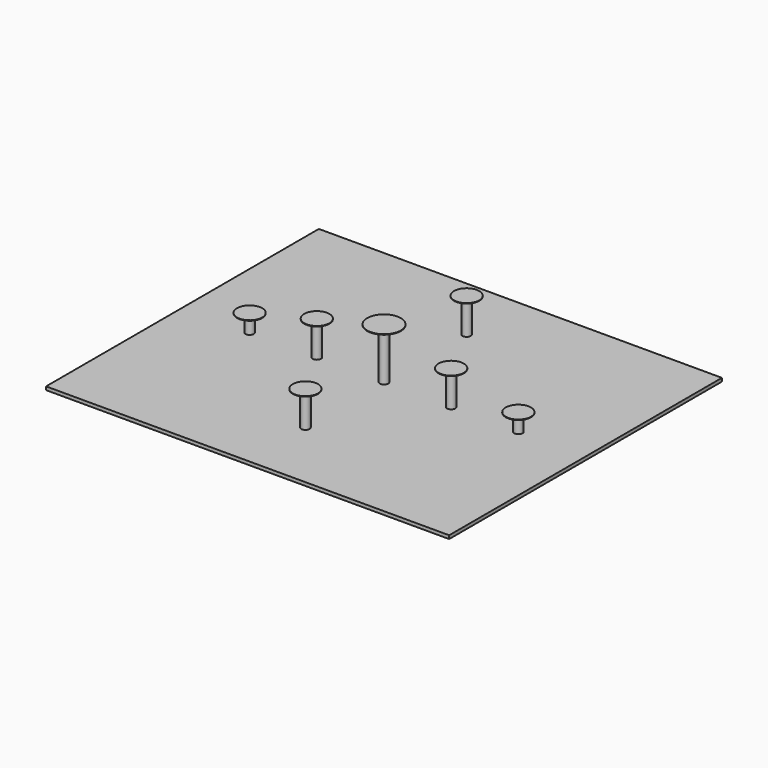
from build123d import *

# Parameters (mm, degrees)
F0_W      = 12000
F0_H      = 100
F1_DEPTH  = 10150
F10_DEPTH = 1500
F11_DEPTH = 500
F12_DEPTH = 1000
F16_DEPTH = 1000
F17_R     = 375
F17_R_2   = 125
F18_DEPTH = 15
F19_R     = 500
F19_R_2   = 125
F20_DEPTH = 15
F21_R     = 375
F21_R_2   = 125
F22_DEPTH = 15
F23_R     = 375
F23_R_2   = 125
F24_DEPTH = 15
F25_R     = 375
F26_DEPTH = 15
F27_R     = 375
F27_R_2   = 125
F28_DEPTH = 15
F29_R     = 375
F29_R_2   = 125
F30_DEPTH = 15


with BuildPart() as f1:
    # F0 (on Front) → F1 (new body)
    with BuildSketch(Plane.XZ):
        with Locations((5386.4197711137, 50)):
            Rectangle(F0_W, F0_H)
    extrude(amount=F1_DEPTH)

    # F3 (on face) → F10 (join)
    with BuildSketch(Plane.XY.offset(100)):
        with BuildLine():
            ThreePointArc((5261.4859178516, -5075), (5386.7112163429, -5199.5475631242), (5511.4850997925, -5074.5477676392))
            ThreePointArc((5511.4850997925, -5074.5477676392), (5474.8503472463, -4986.136325832), (5386.4197711137, -4949.5477847105))
            Line((5386.4197711137, -4949.5477847105), (5386.4197711137, -5075))
            Line((5386.4197711137, -5075), (5261.4859178516, -5075))
        make_face()
        with BuildLine():
            Line((5386.4197711137, -5075), (5386.4197711137, -4949.5477847105))
            ThreePointArc((5386.4197711137, -4949.5477847105), (5297.9139558776, -4986.3425950833), (5261.4859178516, -5075))
            Line((5261.4859178516, -5075), (5386.4197711137, -5075))
        make_face()
    extrude(amount=F10_DEPTH)

    # F14 (on face) + F15 (on face) → F16 (join)
    with BuildSketch(Plane.XY.offset(100)):
        with BuildLine():
            Line((5386.4197711137, -2124.6855282454), (5386.4197711137, -1874.6862387986))
            ThreePointArc((5386.4197711137, -1874.6862387986), (5261.7177963257, -1999.685883522), (5386.4197711137, -2124.6855282454))
        make_face()
        with BuildLine():
            ThreePointArc((5386.4197711137, -2124.6855282454), (5475.0007132703, -2088.1795362647), (5511.7177963257, -1999.685883522))
            ThreePointArc((5511.7177963257, -1999.685883522), (5475.0007132703, -1911.1922307793), (5386.4197711137, -1874.6862387986))
            Line((5386.4197711137, -1874.6862387986), (5386.4197711137, -2124.6855282454))
        make_face()
    with BuildSketch(Plane.XY.offset(100)):
        with BuildLine():
            Line((5386.4197711137, -8124.6809841205), (5386.4197711137, -7874.6810077618))
            ThreePointArc((5386.4197711137, -7874.6810077618), (5261.4741325378, -7999.6809959412), (5386.4197711137, -8124.6809841205))
        make_face()
        with BuildLine():
            ThreePointArc((5386.4197711137, -8124.6809841205), (5474.8432584303, -8088.0885611661), (5511.4741325378, -7999.6809959412))
            ThreePointArc((5511.4741325378, -7999.6809959412), (5474.8432584303, -7911.2734307162), (5386.4197711137, -7874.6810077618))
            Line((5386.4197711137, -7874.6810077618), (5386.4197711137, -8124.6809841205))
        make_face()
    extrude(amount=F16_DEPTH)

    # F17 (on face) → F18 (join)
    with BuildSketch(Plane.XY.offset(1100)):
        with Locations((5386.7177963257, -1999.685883522)):
            Circle(F17_R)
        with Locations((5386.7177963257, -1999.685883522)):
            Circle(F17_R_2, mode=Mode.SUBTRACT)
        with Locations((5386.7177963257, -1999.685883522)):
            Circle(F17_R_2)
    extrude(amount=F18_DEPTH)

    # F19 (on face) → F20 (join)
    with BuildSketch(Plane.XY.offset(1600)):
        with Locations((5386.4850997925, -5074.5477676392)):
            Circle(F19_R)
        with Locations((5386.4850997925, -5074.5477676392)):
            Circle(F19_R_2, mode=Mode.SUBTRACT)
        with Locations((5386.4850997925, -5074.5477676392)):
            Circle(F19_R_2)
    extrude(amount=F20_DEPTH)


with BuildPart() as f11:
    # F9 (on face) → F11 (new body)
    with BuildSketch(Plane.XY.offset(100)):
        with BuildLine():
            ThreePointArc((1261.4053853762, -5075), (1386.3575220073, -5200.0956443843), (1511.4053487778, -5075.0956535339))
            ThreePointArc((1511.4053487778, -5075.0956535339), (1474.7987953448, -4986.7124050985), (1386.4197711137, -4950.095654366))
            Line((1386.4197711137, -4950.095654366), (1386.4197711137, -5075))
            Line((1386.4197711137, -5075), (1261.4053853762, -5075))
        make_face()
        with BuildLine():
            Line((1386.4197711137, -5075), (1386.4197711137, -4950.095654366))
            ThreePointArc((1386.4197711137, -4950.095654366), (1298.0559273963, -4986.6683967543), (1261.4053853762, -5075))
            Line((1261.4053853762, -5075), (1386.4197711137, -5075))
        make_face()
    extrude(amount=F11_DEPTH)

    # F23 (on face) → F24 (join)
    with BuildSketch(Plane.XY.offset(600)):
        with Locations((1386.4053487778, -5075.0956535339)):
            Circle(F23_R)
        with Locations((1386.4053487778, -5075.0956535339)):
            Circle(F23_R_2, mode=Mode.SUBTRACT)
        with Locations((1386.4053487778, -5075.0956535339)):
            Circle(F23_R_2)
    extrude(amount=F24_DEPTH)


with BuildPart() as f11b:
    # F7 (on face) → F11, piece 2 (new body)
    with BuildSketch(Plane.XY.offset(100)):
        with BuildLine():
            ThreePointArc((9261.384189125, -5075), (9386.4897251507, -5199.7885257015), (9511.3840103149, -5074.7885704041))
            ThreePointArc((9511.3840103149, -5074.7885704041), (9474.7850004108, -4986.4128670118), (9386.4197711137, -4949.7885755194))
            Line((9386.4197711137, -4949.7885755194), (9386.4197711137, -5075))
            Line((9386.4197711137, -5075), (9261.384189125, -5075))
        make_face()
        with BuildLine():
            Line((9386.4197711137, -5075), (9386.4197711137, -4949.7885755194))
            ThreePointArc((9386.4197711137, -4949.7885755194), (9297.9335761584, -4986.462352906), (9261.384189125, -5075))
            Line((9261.384189125, -5075), (9386.4197711137, -5075))
        make_face()
    extrude(amount=F11_DEPTH)

    # F29 (on face) → F30 (join)
    with BuildSketch(Plane.XY.offset(600)):
        with Locations((9386.3840103149, -5074.7885704041)):
            Circle(F29_R)
        with Locations((9386.3840103149, -5074.7885704041)):
            Circle(F29_R_2, mode=Mode.SUBTRACT)
        with Locations((9386.3840103149, -5074.7885704041)):
            Circle(F29_R_2)
    extrude(amount=F30_DEPTH)


with BuildPart() as f12:
    # F8 (on face) → F12 (new body)
    with BuildSketch(Plane.XY.offset(100)):
        with BuildLine():
            Line((3261.397186533, -5075), (3511.3970601406, -5075))
            ThreePointArc((3511.3970601406, -5075), (3386.3971233368, -4950.1256942749), (3261.397186533, -5075))
        make_face()
        with BuildLine():
            ThreePointArc((3261.397186533, -5075), (3386.3342761914, -5200.1256784758), (3511.3971233368, -5075.1256942749))
            ThreePointArc((3511.3971233368, -5075.1256942749), (3511.3971075377, -5075.0628471295), (3511.3970601406, -5075))
            Line((3511.3970601406, -5075), (3261.397186533, -5075))
        make_face()
    extrude(amount=F12_DEPTH)

    # F25 (on face) → F26 (join)
    with BuildSketch(Plane.XY.offset(1100)):
        with Locations((3386.3971233368, -5075.1256942749)):
            Circle(F25_R)
        with BuildLine():
            ThreePointArc((3511.3971233368, -5075.1256942749), (3261.3971391358, -5075.1885414211), (3511.3970601406, -5075))
            ThreePointArc((3511.3970601406, -5075), (3511.3971075377, -5075.0628471295), (3511.3971233368, -5075.1256942749))
        make_face(mode=Mode.SUBTRACT)
        with BuildLine():
            ThreePointArc((3511.3971233368, -5075.1256942749), (3511.3971075377, -5075.0628471295), (3511.3970601406, -5075))
            ThreePointArc((3511.3970601406, -5075), (3261.3971391358, -5075.1885414211), (3511.3971233368, -5075.1256942749))
        make_face()
    extrude(amount=F26_DEPTH)


with BuildPart() as f12b:
    # F6 (on face) → F12, piece 2 (new body)
    with BuildSketch(Plane.XY.offset(100)):
        with BuildLine():
            ThreePointArc((7261.3601987157, -5075), (7386.4036560085, -5199.9130173377), (7511.360168457, -5074.9130249023))
            ThreePointArc((7511.360168457, -5074.9130249023), (7474.7695863153, -4986.545752488), (7386.4197711137, -4949.9130391123))
            Line((7386.4197711137, -4949.9130391123), (7386.4197711137, -5075))
            Line((7386.4197711137, -5075), (7261.3601987157, -5075))
        make_face()
        with BuildLine():
            Line((7386.4197711137, -5075), (7386.4197711137, -4949.9130391123))
            ThreePointArc((7386.4197711137, -4949.9130391123), (7297.9621437175, -4986.5343554048), (7261.3601987157, -5075))
            Line((7261.3601987157, -5075), (7386.4197711137, -5075))
        make_face()
    extrude(amount=F12_DEPTH)

    # F27 (on face) → F28 (join)
    with BuildSketch(Plane.XY.offset(1100)):
        with Locations((7386.360168457, -5074.9130249023)):
            Circle(F27_R)
        with Locations((7386.360168457, -5074.9130249023)):
            Circle(F27_R_2, mode=Mode.SUBTRACT)
        with Locations((7386.360168457, -5074.9130249023)):
            Circle(F27_R_2)
    extrude(amount=F28_DEPTH)


with BuildPart() as f22:
    # F21 (on face) → F22 (new body)
    with BuildSketch(Plane.XY.offset(1100)):
        with Locations((5386.4741325378, -7999.6809959412)):
            Circle(F21_R)
        with Locations((5386.4741325378, -7999.6809959412)):
            Circle(F21_R_2, mode=Mode.SUBTRACT)
        with Locations((5386.4741325378, -7999.6809959412)):
            Circle(F21_R_2)
    extrude(amount=F22_DEPTH)


solid = Compound([f1.part, f11.part, f11b.part, f12.part, f12b.part, f22.part])
